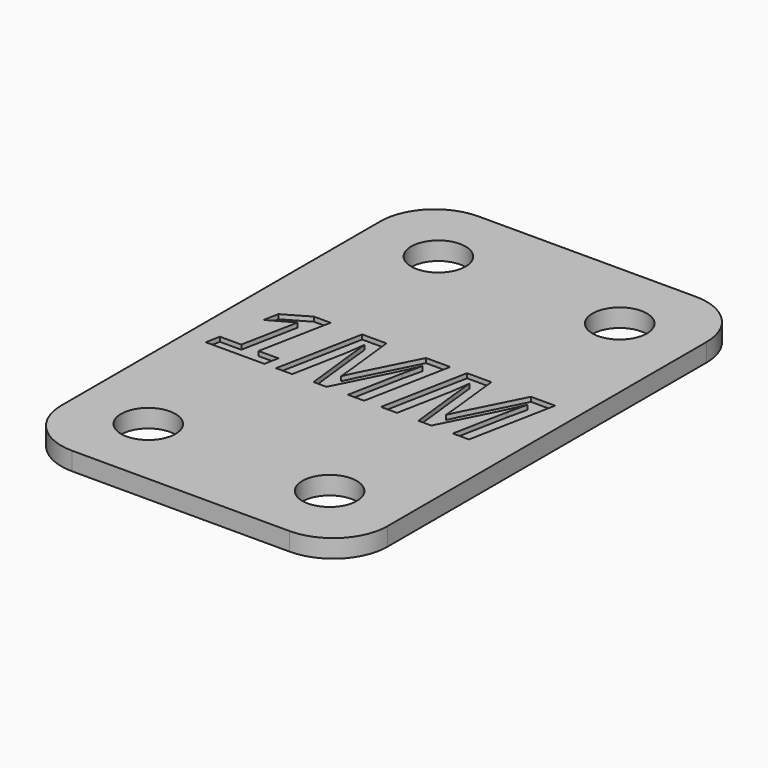
from build123d import *

# Parameters (mm, degrees)
F0_W         = 18
F0_H         = 28
F0_R         = 1.5
F1_DEPTH     = 1
F2_R         = 3
F3_TEXT_SIZE = 6.9444444444
F4_DEPTH     = 0.25


# Not quite as in the source:
# - Text() gives the source's letters only with a copy of the font that has no kerning and outlines rounded to 1/6400 em; it was checked with that copy


with BuildPart() as f1:
    # F0 (on Top) → F1 (new body)
    with BuildSketch(Plane.XY):
        with Locations((-46.9348277748, 3.2886741219)):
            Rectangle(F0_W, F0_H)
        with Locations((-51.9348277748, -6.7113258781)):
            Circle(F0_R, mode=Mode.SUBTRACT)
        with Locations((-41.9348277748, -6.7113258781)):
            Circle(F0_R, mode=Mode.SUBTRACT)
        with Locations((-51.9348277748, 13.2886741219)):
            Circle(F0_R, mode=Mode.SUBTRACT)
        with Locations((-41.9348277748, 13.2886741219)):
            Circle(F0_R, mode=Mode.SUBTRACT)
    extrude(amount=F1_DEPTH)

    # F2
    f2_edges = [f1.edges().sort_by_distance(p)[0] for p in [
        (-37.934828, -10.711326, 0.5),
        (-37.934828, 17.288674, 0.5),
        (-55.934828, 17.288674, 0.5),
        (-55.934828, -10.711326, 0.5),
    ]]
    fillet(f2_edges, radius=F2_R)

    # F3 (on face) → F4 (cut)
    with BuildSketch(Plane.XY.offset(1)):
        with Locations((-54.8722030691, 0.786225711)):
            Text('1MM', F3_TEXT_SIZE, font='Arimo', font_style=FontStyle.BOLDITALIC, text_align=(TextAlign.LEFT, TextAlign.BOTTOM))
    extrude(amount=-F4_DEPTH, mode=Mode.SUBTRACT)


solid = f1.part
